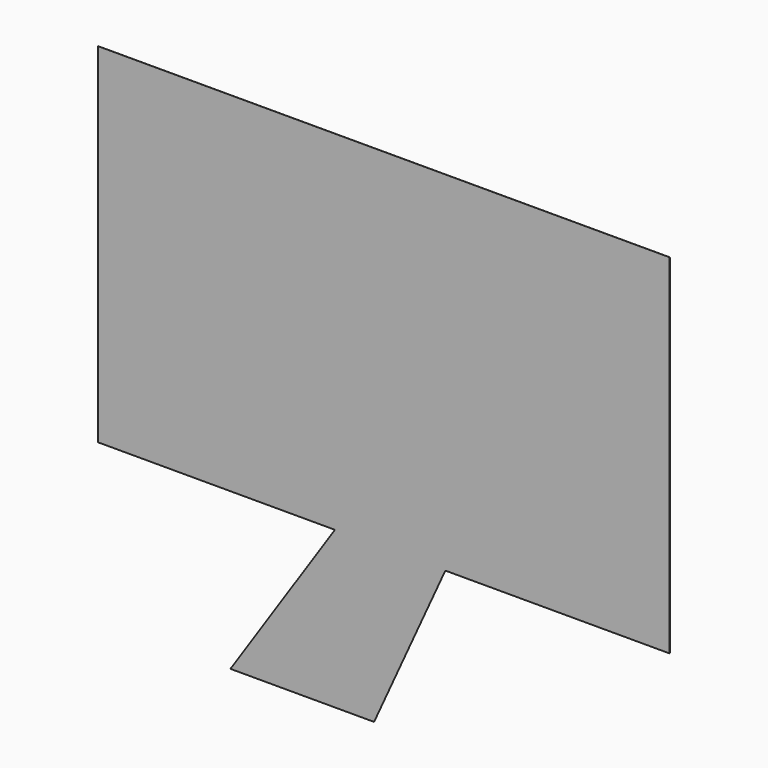
from build123d import *

# Parameters (mm, degrees)
F1_DEPTH     = 2.54
F2_T1_DEPTH  = 116.3302767053
F2_T3_DEPTH  = 79.5286740138
F2_T5_DEPTH  = 45.6964583098
F2_T10_DEPTH = 61.1019260212
F2_T15_DEPTH = 53.0222754018
F2_T20_DEPTH = 50.3447363809
F2_T25_DEPTH = 59.0101457163
F2_T31_DEPTH = 50.1034033931
F2_T35_DEPTH = 53.0222754018
F2_T42_DEPTH = 50.3447363809
F2_T46_DEPTH = 48.0116230882


# Not quite as in the source:
# - a fillet or chamfer that OpenCascade refuses, or shapes differently, is made with other operations: its cross-section is extruded or revolved along the edge and cut away or added


with BuildPart() as f1:
    # F0 (on Front) → F1 (new body)
    with BuildSketch(Plane.XZ):
        Polygon((67.8614974022, 19.1138908267), (-26.4717340469, 19.1138908267), (-26.4717340469, -38.417737931), (12.6331467181, -38.417737931), (30.848396942, -38.417737931), (67.8614974022, -38.417737931), align=None)
        Polygon((30.848396942, -38.417737931), (12.6331467181, -38.417737931), (-4.6027889475, -64.2147809267), (19.0966241062, -64.2147809267), align=None)
    extrude(amount=F1_DEPTH)

    # F2: fillet of radius 5.08 on 8 edges, made by hand

    # F2_s2 → F2_t1 (cut)
    with BuildSketch(Plane.YZ.offset(-37.470256675)):
        with BuildLine():
            ThreePointArc((-2.54, 19.1138908267), (-0.6805909488, 17.2544817755), (0, 14.7144817755))
            Line((0, 14.7144817755), (0, 19.1138908267))
            Line((0, 19.1138908267), (-2.54, 19.1138908267))
        make_face()
    extrude(amount=F2_T1_DEPTH, mode=Mode.SUBTRACT)

    # F2_s4 → F2_t3 (cut)
    with BuildSketch(Plane.XY.offset(-49.4162605591)):
        with BuildLine():
            ThreePointArc((-26.4717340469, -2.54), (-24.6123249957, -0.6805909488), (-22.0723249957, 0))
            Line((-22.0723249957, 0), (-26.4717340469, 0))
            Line((-26.4717340469, 0), (-26.4717340469, -2.54))
        make_face()
        with BuildLine():
            ThreePointArc((67.8614974022, -2.54), (66.002088351, -0.6805909488), (63.462088351, 0))
            Line((63.462088351, 0), (67.8614974022, 0))
            Line((67.8614974022, 0), (67.8614974022, -2.54))
        make_face()
    extrude(amount=F2_T3_DEPTH, mode=Mode.SUBTRACT)

    # F2_s6 → F2_t5 (cut)
    with BuildSketch(Plane.YZ.offset(-15.6013115756)):
        with BuildLine():
            ThreePointArc((-2.54, -64.2147809267), (-0.6805909488, -62.3553718755), (0, -59.8153718755))
            Line((0, -59.8153718755), (0, -64.2147809267))
            Line((0, -64.2147809267), (-2.54, -64.2147809267))
        make_face()
    extrude(amount=F2_T5_DEPTH, mode=Mode.SUBTRACT)


with BuildPart() as f2_tool8:
    # F2_s9 → F2_t10 (new body)
    with BuildSketch(Plane.YZ.offset(-37.470256675)):
        with BuildLine():
            ThreePointArc((-2.54, -38.417737931), (-0.6805909488, -36.5583288798), (0, -34.0183288798))
            Line((0, -34.0183288798), (0, -38.417737931))
            Line((0, -38.417737931), (-2.54, -38.417737931))
        make_face()
    extrude(amount=F2_T10_DEPTH)

    split(bisect_by=Plane(origin=(26.480413057, 0, -17.6925198724), x_dir=(0, 1, 0), z_dir=(-0.8314859511, 0, 0.5555457795)), keep=Keep.TOP)


with BuildPart() as f1_1:
    add(f1.part)

    # F2_t7: cut F2_tool8
    add(f2_tool8.part, mode=Mode.SUBTRACT)


with BuildPart() as f2_tool13:
    # F2_s14 → F2_t15 (new body)
    with BuildSketch(Plane(origin=(-7.737083512, 0, -11.5801010106), x_dir=(0, 1, 0), z_dir=(-0.5555457795, 0, -0.8314859511))):
        with BuildLine():
            ThreePointArc((-2.54, 31.8470961801), (-0.6805909488, 33.7065052313), (0, 36.2465052313))
            Line((0, 36.2465052313), (0, 31.8470961801))
            Line((0, 31.8470961801), (-2.54, 31.8470961801))
        make_face()
    extrude(amount=F2_T15_DEPTH)

    split(bisect_by=Plane.XY.offset(-38.417737931), keep=Keep.BOTTOM)


with BuildPart() as f1_2:
    add(f1_1.part)

    # F2_t12: cut F2_tool13
    add(f2_tool13.part, mode=Mode.SUBTRACT)


with BuildPart() as f2_tool18:
    # F2_s19 → F2_t20 (new body)
    with BuildSketch(Plane(origin=(-25.5031201264, 0, -55.983475482), x_dir=(0, 1, 0), z_dir=(0.4145583774, 0, 0.9100227204))):
        with BuildLine():
            ThreePointArc((-2.54, -43.9991372067), (-0.6805909488, -42.1397281555), (0, -39.5997281555))
            Line((0, -39.5997281555), (0, -43.9991372067))
            Line((0, -43.9991372067), (-2.54, -43.9991372067))
        make_face()
    extrude(amount=F2_T20_DEPTH)

    split(bisect_by=Plane.XY.offset(-38.417737931), keep=Keep.BOTTOM)


with BuildPart() as f1_3:
    add(f1_2.part)

    # F2_t17: cut F2_tool18
    add(f2_tool18.part, mode=Mode.SUBTRACT)


with BuildPart() as f2_tool23:
    # F2_s24 → F2_t25 (new body)
    with BuildSketch(Plane.YZ.offset(19.849874314)):
        with BuildLine():
            ThreePointArc((-2.54, -38.417737931), (-0.6805909488, -36.5583288798), (0, -34.0183288798))
            Line((0, -34.0183288798), (0, -38.417737931))
            Line((0, -38.417737931), (-2.54, -38.417737931))
        make_face()
    extrude(amount=F2_T25_DEPTH)

    split(bisect_by=Plane(origin=(40.040214538, 0, -18.2402109276), x_dir=(0, 1, 0), z_dir=(0.9100227204, 0, -0.4145583774)), keep=Keep.TOP)


with BuildPart() as f1_4:
    add(f1_3.part)

    # F2_t22: cut F2_tool23
    add(f2_tool23.part, mode=Mode.SUBTRACT)


with BuildPart() as f2_tool29:
    # F2_s30 → F2_t31 (new body)
    with BuildSketch(Plane.YZ.offset(-26.4717340469)):
        with BuildLine():
            ThreePointArc((-2.54, -38.417737931), (-0.6805909488, -36.5583288798), (0, -34.0183288798))
            Line((0, -34.0183288798), (0, -38.417737931))
            Line((0, -38.417737931), (-2.54, -38.417737931))
        make_face()
    extrude(amount=F2_T31_DEPTH)

    split(bisect_by=Plane(origin=(26.480413057, 0, -17.6925198724), x_dir=(0, 1, 0), z_dir=(0.8314859511, 0, -0.5555457795)), keep=Keep.TOP)


with BuildPart() as f2_tool33:
    # F2_s34 → F2_t35 (new body)
    with BuildSketch(Plane(origin=(-7.737083512, 0, -11.5801010106), x_dir=(0, 1, 0), z_dir=(-0.5555457795, 0, -0.8314859511))):
        with BuildLine():
            ThreePointArc((-2.54, 31.8470961801), (-0.6805909488, 33.7065052313), (0, 36.2465052313))
            Line((0, 36.2465052313), (0, 31.8470961801))
            Line((0, 31.8470961801), (-2.54, 31.8470961801))
        make_face()
    extrude(amount=F2_T35_DEPTH)

    split(bisect_by=Plane.XY.offset(-38.417737931), keep=Keep.TOP)


with BuildPart() as f2_tool29_1:
    add(f2_tool29.part)

    # F2_t37: intersect F2_tool33
    add(f2_tool33.part, mode=Mode.INTERSECT)


with BuildPart() as f1_5:
    add(f1_4.part)

    # F2_t27: cut F2_tool29
    add(f2_tool29_1.part, mode=Mode.SUBTRACT)


with BuildPart() as f2_tool40:
    # F2_s41 → F2_t42 (new body)
    with BuildSketch(Plane(origin=(-25.5031201264, 0, -55.983475482), x_dir=(0, 1, 0), z_dir=(0.4145583774, 0, 0.9100227204))):
        with BuildLine():
            ThreePointArc((-2.54, -43.9991372067), (-0.6805909488, -42.1397281555), (0, -39.5997281555))
            Line((0, -39.5997281555), (0, -43.9991372067))
            Line((0, -43.9991372067), (-2.54, -43.9991372067))
        make_face()
    extrude(amount=F2_T42_DEPTH)

    split(bisect_by=Plane.XY.offset(-38.417737931), keep=Keep.TOP)


with BuildPart() as f2_tool44:
    # F2_s45 → F2_t46 (new body)
    with BuildSketch(Plane.YZ.offset(19.849874314)):
        with BuildLine():
            ThreePointArc((-2.54, -38.417737931), (-0.6805909488, -36.5583288798), (0, -34.0183288798))
            Line((0, -34.0183288798), (0, -38.417737931))
            Line((0, -38.417737931), (-2.54, -38.417737931))
        make_face()
    extrude(amount=F2_T46_DEPTH)

    split(bisect_by=Plane(origin=(40.040214538, 0, -18.2402109276), x_dir=(0, 1, 0), z_dir=(-0.9100227204, 0, 0.4145583774)), keep=Keep.TOP)


with BuildPart() as f2_tool40_1:
    add(f2_tool40.part)

    # F2_t48: intersect F2_tool44
    add(f2_tool44.part, mode=Mode.INTERSECT)


with BuildPart() as f1_6:
    add(f1_5.part)

    # F2_t38: cut F2_tool40
    add(f2_tool40_1.part, mode=Mode.SUBTRACT)


solid = f1_6.part
